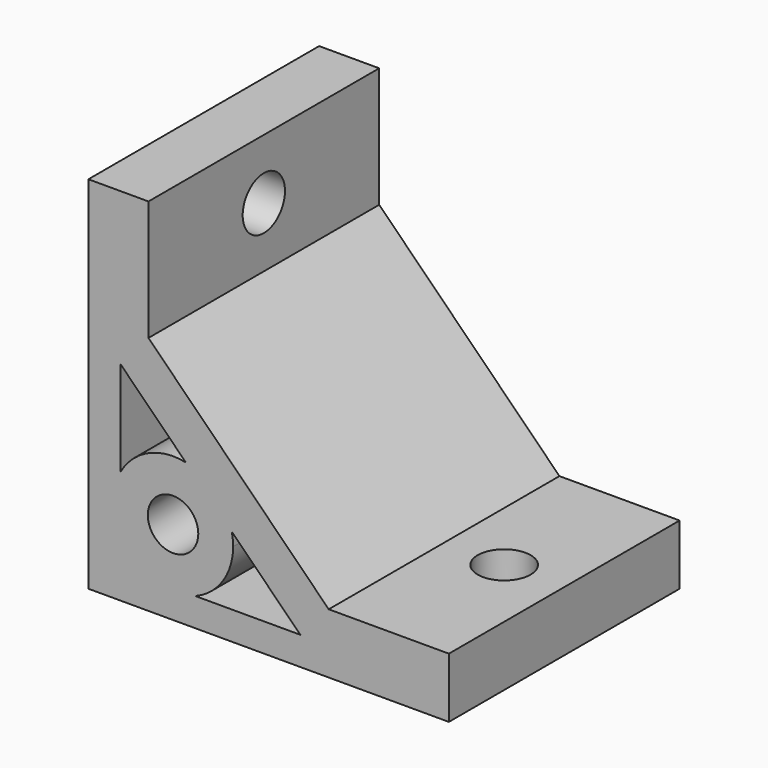
from build123d import *

# Parameters (mm, degrees)
F1_W     = 8
F1_H     = 30
F1_R     = 2.2
F2_DEPTH = 5
F0_W     = 30
F0_H     = 8
F0_R     = 2.2
F3_DEPTH = 5
F5_SIZE  = 15
F4_R     = 2.1
F6_DEPTH = 30


with BuildPart() as f2:
    # F1 (on Right) → F2 (new body)
    with BuildSketch(Plane.YZ):
        with Locations((20, 15)):
            Rectangle(F1_W, F1_H)
        with Locations((12, 15)):
            Rectangle(F1_W, F1_H)
        with Locations((12.000000596, 25)):
            Circle(F1_R, mode=Mode.SUBTRACT)
        with Locations((4, 15)):
            Rectangle(F1_W, F1_H)
    extrude(amount=F2_DEPTH)

    # F0 (on Top) → F3 (join)
    with BuildSketch(Plane.XY):
        with Locations((15, 20)):
            Rectangle(F0_W, F0_H)
        with Locations((15, 12)):
            Rectangle(F0_W, F0_H)
        with Locations((25, 12)):
            Circle(F0_R, mode=Mode.SUBTRACT)
        with Locations((15, 4)):
            Rectangle(F0_W, F0_H)
    extrude(amount=F3_DEPTH)

    # F5
    f5_edges = [f2.edges().sort_by_distance(p)[0] for p in [
        (5, 12, 5),
    ]]
    chamfer(f5_edges, length=F5_SIZE)

    # F4 (on Front) → F6 (cut)
    with BuildSketch(Plane.XZ):
        with BuildLine():
            Line((8.9047972998, 2.3616264964), (17.6383735036, 2.3616264964))
            Line((17.6383735036, 2.3616264964), (11.929701132, 8.070298868))
            ThreePointArc((11.929701132, 8.070298868), (12.0160710439, 7.5396825646), (12.0449723862, 7.0028603077))
            ThreePointArc((12.0449723862, 7.0028603077), (11.1861753858, 4.2009970498), (8.9047972998, 2.3616264964))
        make_face()
        with BuildLine():
            ThreePointArc((2.6568189153, 9.3995474202), (4.970273692, 11.5521047865), (8.1124109465, 11.8875890535))
            Line((8.1124109465, 11.8875890535), (2.6568189153, 17.3431810847))
            Line((2.6568189153, 17.3431810847), (2.6568189153, 9.3995474202))
        make_face()
        with Locations((7.0449723862, 7.0028603077)):
            Circle(F4_R)
    extrude(amount=-F6_DEPTH, mode=Mode.SUBTRACT)


solid = f2.part
